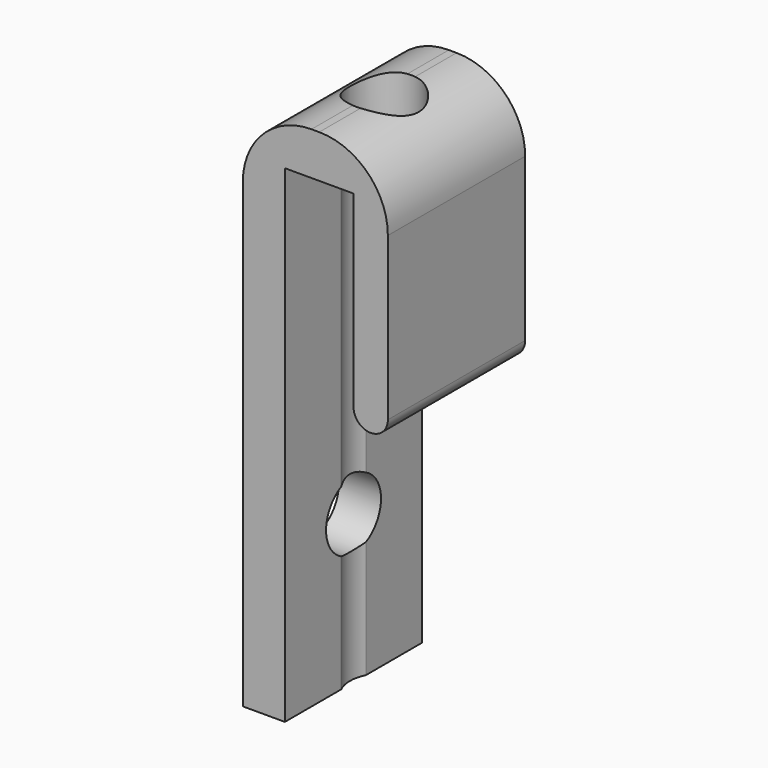
from build123d import *

# Parameters (mm, degrees)
F1_DEPTH = 6.35
F2_R     = 5.08
F5_D     = 5.08
F6_D     = 5.08
F7_R     = 1.26999


# Not quite as in the source:
# - a fillet or chamfer is up to 0.001 mm smaller than in the source, because OpenCascade refuses the exact size


with BuildPart() as f1:
    # F0 (on Front) → F1 (new body, symmetric)
    with BuildSketch(Plane.XZ):
        Polygon((-2.54, 0), (0, 0), (0, 18.3514992646), (-10.7314998529, 18.3514992646), (-10.7314998529, -20.8914992646), (-7.62, -20.8914992646), (-7.62, 15.176498382), (-2.54, 15.176498382), align=None)
    extrude(amount=F1_DEPTH, both=True)

    # F2
    f2_edges = [f1.edges().sort_by_distance(p)[0] for p in [
        (0, 0, 18.351499),
        (-10.7315, 0, 18.351499),
    ]]
    fillet(f2_edges, radius=F2_R)

    # F5 (through all)
    with Locations(Plane.XY.offset(18.3514992646)):
        with Locations((-5.3486400284, 0)):
            Hole(F5_D / 2)

    # F6 (through all)
    with Locations(Plane(origin=(-10.7314998529, 0, 0), x_dir=(0, -1, 0), z_dir=(-1, 0, 0))):
        with Locations((0, -9.9572697654)):
            Hole(F6_D / 2)

    # F7 (radius 1.27 in the source; OpenCascade refuses exactly that, so slightly less here)
    f7_edges = [f1.edges().sort_by_distance(p)[0] for p in [
        (0, 0, 0),
        (-2.54, 0, 0),
    ]]
    fillet(f7_edges, radius=F7_R)


solid = f1.part
